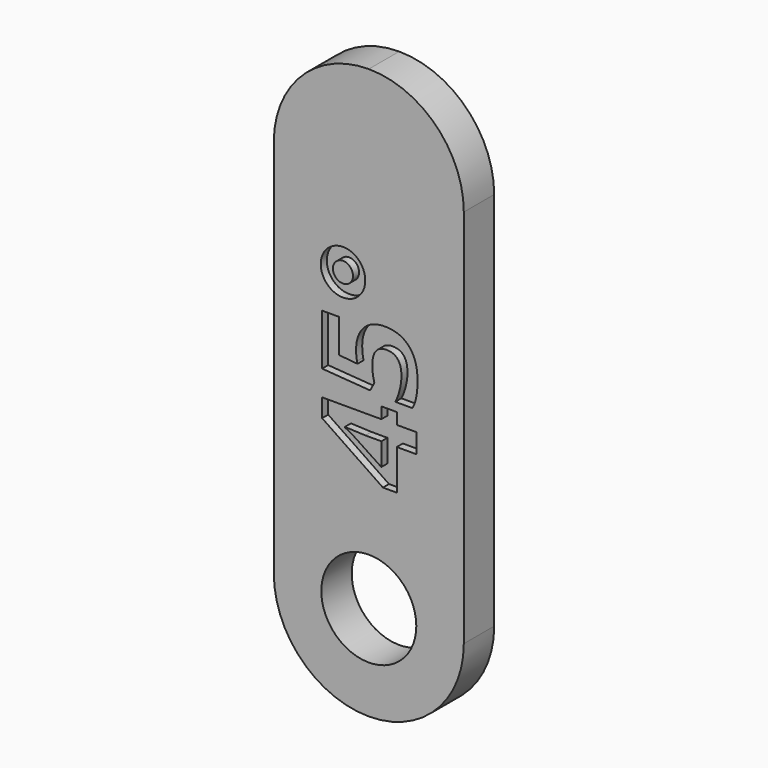
from build123d import *

# Parameters (mm, degrees)
F0_W         = 12.7
F0_H         = 38.1
F0_R         = 3.175
F1_DEPTH     = 2.54
F2_R         = 6.34999
F3_TEXT_SIZE = 8.8194444444
F4_DEPTH     = 0.508


# Not quite as in the source:
# - a fillet or chamfer is up to 0.001 mm smaller than in the source, because OpenCascade refuses the exact size
# - Text() gives the source's letters only with a copy of the font that has no kerning and outlines rounded to 1/6400 em; it was checked with that copy


with BuildPart() as f1:
    # F0 (on Front) → F1 (new body)
    with BuildSketch(Plane.XZ):
        with Locations((6.35, 19.05)):
            Rectangle(F0_W, F0_H)
        with Locations((6.35, 6.35)):
            Circle(F0_R, mode=Mode.SUBTRACT)
    extrude(amount=F1_DEPTH)

    # F2 (radius 6.35 in the source; OpenCascade refuses exactly that, so slightly less here)
    f2_edges = [f1.edges().sort_by_distance(p)[0] for p in [
        (12.7, -1.27, 0),
        (0, -1.27, 0),
        (12.7, -1.27, 38.1),
        (0, -1.27, 38.1),
    ]]
    fillet(f2_edges, radius=F2_R)

    # F3 (on face) → F4 (cut)
    with BuildSketch(Plane.XZ.offset(2.54)):
        with Locations(Location((9.525, 13.6294867622), (0, 0, 90))):
            Text('45°', F3_TEXT_SIZE, font='Open Sans', font_style=FontStyle.BOLD, text_align=(TextAlign.LEFT, TextAlign.BOTTOM))
    extrude(amount=-F4_DEPTH, mode=Mode.SUBTRACT)


solid = f1.part
